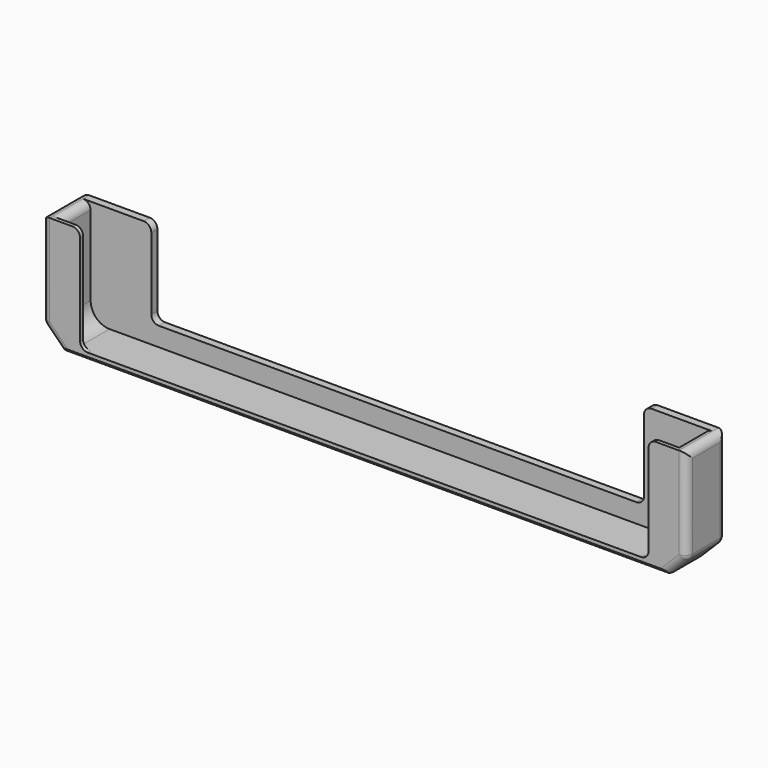
from build123d import *

# Parameters (mm, degrees)
F0_W     = 170
F0_H     = 30
F1_DEPTH = 13
F3_DEPTH = 28
F4_W     = 130
F4_H     = 2
F5_DEPTH = 5
F6_SIZE  = 5
F7_R     = 5
F8_SIZE  = 1
F9_R     = 1.99999


# Not quite as in the source:
# - a fillet or chamfer is up to 0.001 mm smaller than in the source, because OpenCascade refuses the exact size


with BuildPart() as f1:
    # F0 (on Front) → F1 (new body)
    with BuildSketch(Plane.XZ):
        with Locations((0, 15)):
            Rectangle(F0_W, F0_H)
    extrude(amount=F1_DEPTH)

    # F2 (on face) → F3 (cut)
    with BuildSketch(Plane.XY.offset(30)):
        Polygon((-65, -2), (-81, -2), (-81, -12), (-75, -12), (-75, -13), (75, -13), (75, -12), (81, -12), (81, -2), (65, -2), (65, 0), (-65, 0), align=None)
    extrude(amount=-F3_DEPTH, mode=Mode.SUBTRACT)

    # F4 (on face) → F5 (join)
    with BuildSketch(Plane.XY.offset(2)):
        with Locations((0, -1)):
            Rectangle(F4_W, F4_H)
    extrude(amount=F5_DEPTH)

    # F6
    f6_edges = [f1.edges().sort_by_distance(p)[0] for p in [
        (85, -6.5, 0),
        (-85, -6.5, 0),
    ]]
    chamfer(f6_edges, length=F6_SIZE)

    # F7
    f7_edges = [f1.edges().sort_by_distance(p)[0] for p in [
        (-81, -7, 2),
        (81, -7, 2),
    ]]
    fillet(f7_edges, radius=F7_R)

    # F8
    f8_edges = [f1.edges().sort_by_distance(p)[0] for p in [
        (0, -13, 0),
        (0, 0, 0),
    ]]
    chamfer(f8_edges, length=F8_SIZE)

    # F9 (radius 2 in the source; OpenCascade refuses exactly that, so slightly less here)
    f9_edges = [f1.edges().sort_by_distance(p)[0] for p in [
        (-85, -6.5, 5),
        (-85, -6.5, 30),
        (-81, -7, 30),
        (81, -7, 30),
        (85, -6.5, 30),
        (85, -6.5, 5),
        (65, -1, 7),
        (65, -1, 30),
        (75, -12.5, 2),
        (75, -12.5, 30),
        (-65, -1, 30),
        (-65, -1, 7),
        (-75, -12.5, 2),
        (-75, -12.5, 30),
        (85, 0, 17.5),
        (83, 0, 3),
        (83, -13, 3),
        (85, -13, 17.5),
        (-85, 0, 17.5),
        (-83, 0, 3),
        (-85, -13, 17.5),
        (-83, -13, 3),
    ]]
    fillet(f9_edges, radius=F9_R)


solid = f1.part
